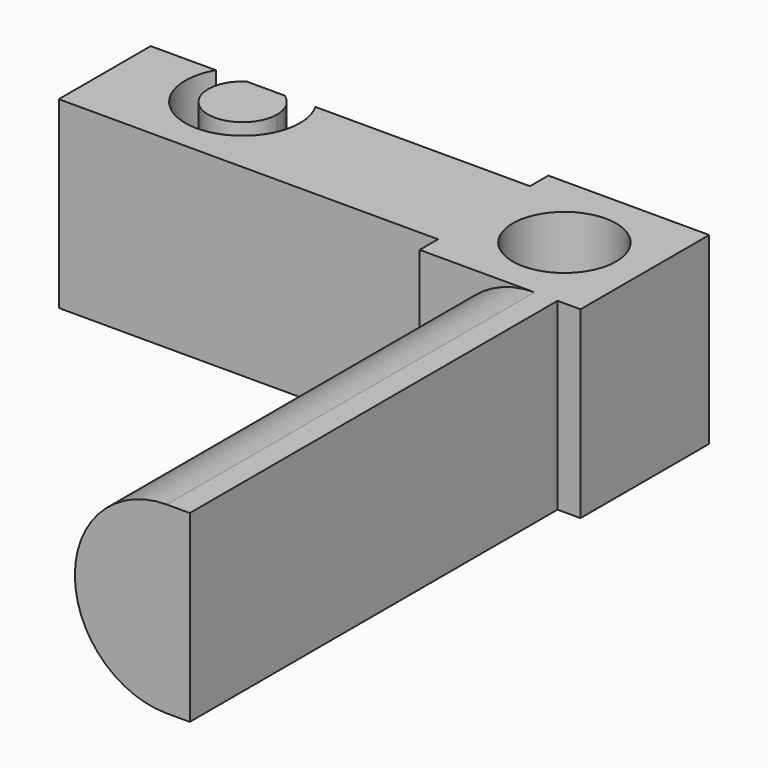
from build123d import *

# Parameters (mm, degrees)
F0_W     = 5
F0_H     = 20
F0_R     = 2.25
F0_W_2   = 16.5
F0_H_2   = 5
F1_DEPTH = 8
F2_R     = 3.99999
F4_DEPTH = 5


# Not quite as in the source:
# - a fillet or chamfer is up to 0.001 mm smaller than in the source, because OpenCascade refuses the exact size
# - a feature names something its author has since deleted; it is built from what else it names


with BuildPart() as f1:
    # F0 (on Top) → F1 (new body)
    with BuildSketch(Plane.XY):
        Rectangle(F0_W, F0_H)
        Polygon((-2.5, 10), (2.5, 10), (3.5, 10), (3.5, 17), (-3.5, 17), (-3.5, 16), (-3.5, 11), (-3.5, 10), align=None)
        with Locations((0, 13.5)):
            Circle(F0_R, mode=Mode.SUBTRACT)
        with Locations((-11.75, 13.5)):
            Rectangle(F0_W_2, F0_H_2)
    extrude(amount=F1_DEPTH)

    # F2 (radius 4 in the source; OpenCascade refuses exactly that, so slightly less here)
    f2_edges = [f1.edges().sort_by_distance(p)[0] for p in [
        (-2.5, 0, 8),
        (-2.5, 0, 0),
    ]]
    fillet(f2_edges, radius=F2_R)

    # F3 (on face) → F4 (cut)
    with BuildSketch(Plane.XY.offset(8)):
        with BuildLine():
            ThreePointArc((-15.8291561976, 16), (-15, 16.25), (-14.1708438024, 16))
            Line((-14.1708438024, 16), (-12.8349364905, 16))
            ThreePointArc((-12.8349364905, 16), (-15, 17.25), (-17.1650635095, 16))
            Line((-17.1650635095, 16), (-15.8291561976, 16))
        make_face()
        with BuildLine():
            ThreePointArc((-14.1708438024, 16), (-13.6783089816, 15.4593185827), (-13.5, 14.75))
            ThreePointArc((-13.5, 14.75), (-15.7093185827, 13.4283089816), (-15.8291561976, 16))
            Line((-15.8291561976, 16), (-17.1650635095, 16))
            ThreePointArc((-17.1650635095, 16), (-15.6470476128, 12.3351854343), (-12.5, 14.75))
            ThreePointArc((-12.5, 14.75), (-12.5851854343, 15.3970476128), (-12.8349364905, 16))
            Line((-12.8349364905, 16), (-14.1708438024, 16))
        make_face()
    extrude(amount=-F4_DEPTH, mode=Mode.SUBTRACT)


solid = f1.part
